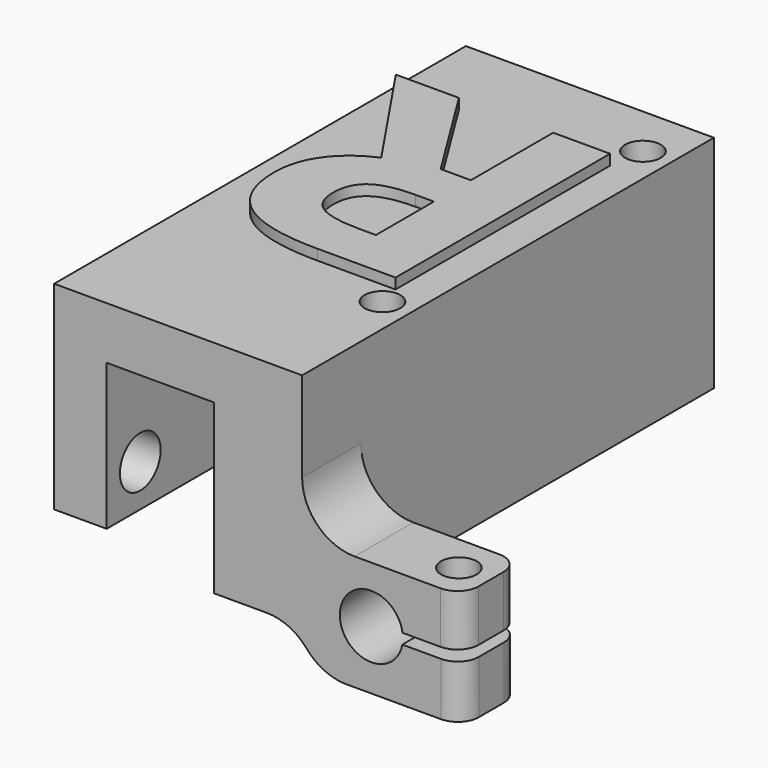
from build123d import *

# Parameters (mm, degrees)
F1_DEPTH      = 7
F2_DEPTH      = 42
F3_R          = 1.7
F3_R_2        = 11
F4_DEPTH      = 21.001
F5_R          = 3
F6_DEPTH      = 10
F7_DEPTH      = 21.001
F8_R          = 1.4
F9_DEPTH      = 11.0176173191
F8_R_2        = 1.7
F10_DEPTH     = 4.91123055
F11_R         = 5
F12_R         = 5
F13_R         = 5
F14_R         = 2
F15_R         = 2.2
F15_R_2       = 2.4255023423
F16_DEPTH     = 6
F17_TEXT_SIZE = 35.7644961357
F18_DEPTH     = 1


# Not quite as in the source:
# - a feature names something its author has since deleted; it is built from what else it names
# - Text() gives the source's letters only with a copy of the font that has no kerning and outlines rounded to 1/6400 em; it was checked with that copy


with BuildPart() as f1:
    # F0 (on Front) → F1 (new body)
    with BuildSketch(Plane.XZ):
        Polygon((-18.6721007523, 29.8099789735), (-18.6721007523, 10.8925135386), (-13.6721007523, 10.8925135386), (-13.6721007523, 24.8099789735), (-3.4721007523, 24.8099789735), (-3.4721007523, 8.8099789735), (4.9380548998, 8.8099789735), (4.9380548998, 16.2656020473), (4.9380548998, 29.8099789735), align=None)
        Polygon((20.1263195603, 16.2417280634), (4.9380548998, 16.2656020473), (4.9380548998, 8.8099789735), (6.3533044869, 5.2860832236), (20.1553367778, 5.2860832236), (20.1553367778, 10.343908232), (13.4860510706, 10.343908232), (13.4860510706, 11.3388913612), (20.1263195603, 11.3388913612), align=None)
    extrude(amount=F1_DEPTH)

    # F0 (on Front) → F2 (join)
    with BuildSketch(Plane.XZ):
        Polygon((-18.6721007523, 29.8099789735), (-18.6721007523, 10.8925135386), (-13.6721007523, 10.8925135386), (-13.6721007523, 24.8099789735), (-3.4721007523, 24.8099789735), (-3.4721007523, 8.8099789735), (4.9380548998, 8.8099789735), (4.9380548998, 16.2656020473), (4.9380548998, 29.8099789735), align=None)
    extrude(amount=-F2_DEPTH)

    # F3 (on face) → F4 (cut, through all)
    with BuildSketch(Plane(origin=(0, 0, 8.8099789735), x_dir=(1, 0, 0), z_dir=(0, 0, -1))):
        with Locations((2.1850741468, -6)):
            Circle(F3_R)
        with Locations((2.1850741468, -37)):
            Circle(F3_R)
        with Locations((17.6850741468, -21.5)):
            Circle(F3_R_2)
    extrude(amount=-F4_DEPTH, mode=Mode.SUBTRACT)

    # F5 (on face) → F6 (cut)
    with BuildSketch(Plane.XZ.offset(7)):
        with Locations((11.5278992477, 10.8989789735)):
            Circle(F5_R)
    extrude(amount=-F6_DEPTH, mode=Mode.SUBTRACT)

    # F3 (on face) → F7 (cut, through all)
    with BuildSketch(Plane(origin=(0, 0, 8.8099789735), x_dir=(1, 0, 0), z_dir=(0, 0, -1))):
        with Locations((2.1850741468, -6)):
            Circle(F3_R)
        with Locations((2.1850741468, -37)):
            Circle(F3_R)
        with Locations((17.6850741468, -21.5)):
            Circle(F3_R_2)
    extrude(amount=-F7_DEPTH, mode=Mode.SUBTRACT)

    # F8 (on face) → F9 (cut, through all)
    with BuildSketch(Plane(origin=(0.0255795563, 0, 16.273323822), x_dir=(0.9999987646, 0, -0.0015718685), z_dir=(0.0015718685, 0, 0.9999987646))):
        with Locations((17.1007648362, -3.5767070949)):
            Circle(F8_R)
    extrude(amount=-F9_DEPTH, mode=Mode.SUBTRACT)

    # F8 (on face) → F10 (cut, through all)
    with BuildSketch(Plane(origin=(0.0255795563, 0, 16.273323822), x_dir=(0.9999987646, 0, -0.0015718685), z_dir=(0.0015718685, 0, 0.9999987646))):
        with Locations((17.1007648362, -3.5767070949)):
            Circle(F8_R_2)
        with Locations((17.1007648362, -3.5767070949)):
            Circle(F8_R, mode=Mode.SUBTRACT)
    extrude(amount=-F10_DEPTH, mode=Mode.SUBTRACT)

    # F11
    f11_edges = [f1.edges().sort_by_distance(p)[0] for p in [
        (4.938055, -3.5, 16.265602),
    ]]
    fillet(f11_edges, radius=F11_R)

    # F12
    f12_edges = [f1.edges().sort_by_distance(p)[0] for p in [
        (4.938055, -3.5, 8.809979),
    ]]
    fillet(f12_edges, radius=F12_R)

    # F13
    f13_edges = [f1.edges().sort_by_distance(p)[0] for p in [
        (6.353304, -3.5, 5.286083),
    ]]
    fillet(f13_edges, radius=F13_R)

    # F14
    f14_edges = [f1.edges().sort_by_distance(p)[0] for p in [
        (20.12632, -7, 13.79031),
        (20.155337, -7, 7.814996),
        (20.12632, 0, 13.79031),
        (20.155337, 0, 7.814996),
    ]]
    fillet(f14_edges, radius=F14_R)

    # F15 (on face) → F16 (cut)
    with BuildSketch(Plane(origin=(-18.6721007523, 0, 0), x_dir=(0, -1, 0), z_dir=(-1, 0, 0))):
        with Locations((-38, 14.8925135386)):
            Circle(F15_R)
        with Locations((3, 14.8925135386)):
            Circle(F15_R_2)
    extrude(amount=-F16_DEPTH, mode=Mode.SUBTRACT)

    # F17 (on face) → F18 (join)
    with BuildSketch(Plane.XY.offset(29.8099789735)):
        with Locations(Location((4.9380548998, 33.6637421799), (0, 0, 180))):
            Text('R', F17_TEXT_SIZE, font='Open Sans', font_style=FontStyle.BOLD, text_align=(TextAlign.LEFT, TextAlign.BOTTOM))
    extrude(amount=F18_DEPTH)


solid = f1.part
